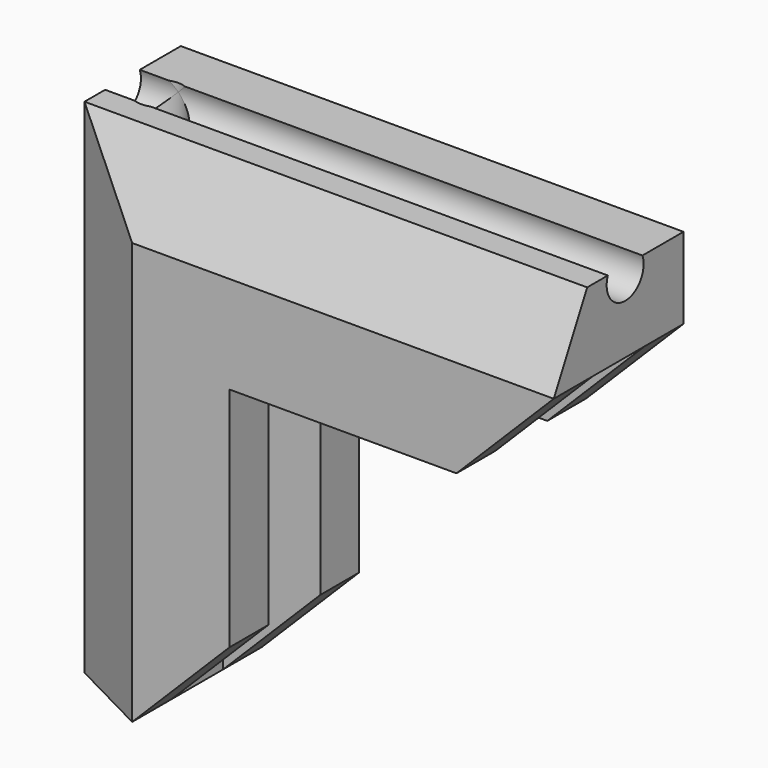
from build123d import *

# Parameters (mm, degrees)
F1_DEPTH      = 20
F2_W          = 7
F2_H          = 20
F3_DEPTH      = 2
F5_DEPTH      = 6
F6_W          = 3
F6_H          = 6
F7_DEPTH      = 25
F8_DEPTH      = 3
F12_DEPTH     = 2
F13_DEPTH     = 11
F14_T4_DEPTH  = 29
F14_T10_DEPTH = 28
F14_T17_DEPTH = 38.2867319519
F14_T24_DEPTH = 39.2867319519
F15_T1_DEPTH  = 61.1449358039
F15_T3_DEPTH  = 60.1449358039
F16_DEPTH     = 1
F17_SIZE      = 6
F20_D         = 2.85
F20_ON_F18_D  = 2.85


# Not quite as in the source:
# - a fillet or chamfer that OpenCascade refuses, or shapes differently, is made with other operations: its cross-section is extruded or revolved along the edge and cut away or added


with BuildPart() as f1:
    # F0 (on Top) → F1 (new body)
    with BuildSketch(Plane.XY):
        Polygon((-3.1551690071, 9.1141472052), (-12.1551690071, 9.1141472052), (-12.1551690071, -0.8858527948), (-3.1551690071, -0.8858527948), (-3.1551690071, 2.1141472052), (-9.1551690071, 2.1141472052), (-9.1551690071, 6.1141472052), (-3.1551690071, 6.1141472052), align=None)
    extrude(amount=F1_DEPTH)

    # F2 (on face) → F3 (join)
    with BuildSketch(Plane(origin=(-12.1551690071, 0, 0), x_dir=(0, -1, 0), z_dir=(-1, 0, 0))):
        with Locations((-5.6141472052, 10)):
            Rectangle(F2_W, F2_H)
    extrude(amount=F3_DEPTH)

    # F4 (on face) → F5 (join)
    with BuildSketch(Plane.XY.offset(20)):
        Polygon((-12.1345976368, 9.1141472052), (-12.1551690071, 2.1141472052), (-12.1551690071, -0.8858527948), (-9.1551690071, -0.8858527948), (-9.1551690071, 2.1141472052), (-9.1551690071, 6.1141472052), (-9.1551690071, 9.1141472052), align=None)
    extrude(amount=F5_DEPTH)

    # F6 (on face) → F7 (join)
    with BuildSketch(Plane.YZ.offset(-9.1551690071)):
        with Locations((7.6141472052, 23)):
            Rectangle(F6_W, F6_H)
        with Locations((0.6141472052, 23)):
            Rectangle(F6_W, F6_H)
        Polygon((-0.8858527948, 26), (2.1141472052, 26), (6.1141472052, 26), (9.1141472052, 26), (9.1141472052, 29), (-0.8858527948, 29), align=None)
    extrude(amount=F7_DEPTH)

    # F8 (add): a face of the model
    f8_faces = [f1.faces().sort_by_distance(p)[0] for p in [
        (-10.6515768532, 4.1077318265, 26),
    ]]
    extrude(f8_faces, amount=F8_DEPTH)

    # F9: union 

    # F10: union 

    # F11 (on face) → F12 (join)
    with BuildSketch(Plane.XY.offset(29)):
        Polygon((-12.1345976368, 9.1141472052), (-12.1551690071, 2.1141472052), (15.8448309929, 2.1141472052), (15.8448309929, 9.1141472052), align=None)
    extrude(amount=F12_DEPTH)

    # F4 (on face) → F13 (join)
    with BuildSketch(Plane.XY.offset(20)):
        Polygon((-14.1551690071, 2.1141472052), (-12.1551690071, 2.1141472052), (-12.1345976368, 9.1141472052), (-14.1551690071, 9.1141472052), align=None)
    extrude(amount=F13_DEPTH)

    # F14: chamfer of 4 on 2 edges, made by hand


with BuildPart() as f14_tool2:
    # F14_s3 → F14_t4 (new body)
    with BuildSketch(Plane.XY):
        Polygon((-12.1551690071, -1.8858527948), (-16.1551690071, 2.1141472052), (-12.1551690071, 2.1141472052), align=None)
    extrude(amount=F14_T4_DEPTH)

    split(bisect_by=Plane.XZ.offset(0.8858527948), keep=Keep.BOTTOM)

    split(bisect_by=Plane.YZ.offset(-14.1551690071), keep=Keep.TOP)


with BuildPart() as f1_1:
    add(f1.part)

    # F14_t1: union F14_tool2
    add(f14_tool2.part)


with BuildPart() as f14_tool8:
    # F14_s9 → F14_t10 (new body)
    with BuildSketch(Plane.YZ.offset(-12.1551690071)):
        Polygon((-1.8858527948, 29), (2.1141472052, 33), (2.1141472052, 29), align=None)
    extrude(amount=F14_T10_DEPTH)

    split(bisect_by=Plane.XZ.offset(0.8858527948), keep=Keep.BOTTOM)

    split(bisect_by=Plane.XY.offset(31), keep=Keep.BOTTOM)


with BuildPart() as f1_2:
    add(f1_1.part)

    # F14_t7: union F14_tool8
    add(f14_tool8.part)


with BuildPart() as f14_tool15:
    # F14_s16 → F14_t17 (new body)
    with BuildSketch(Plane.YZ.offset(-22.4419009589)):
        Polygon((-1.8858527948, 29), (2.1141472052, 33), (2.1141472052, 29), align=None)
    extrude(amount=F14_T17_DEPTH)

    split(bisect_by=Plane.XZ.offset(0.8858527948), keep=Keep.BOTTOM)

    split(bisect_by=Plane.YZ.offset(-12.1551690071), keep=Keep.BOTTOM)

    split(bisect_by=Plane.YZ.offset(-14.1551690071), keep=Keep.TOP)

    split(bisect_by=Plane.XY.offset(31), keep=Keep.BOTTOM)


with BuildPart() as f14_tool22:
    # F14_s23 → F14_t24 (new body)
    with BuildSketch(Plane.XY):
        Polygon((-12.1551690071, -1.8858527948), (-16.1551690071, 2.1141472052), (-12.1551690071, 2.1141472052), align=None)
    extrude(amount=F14_T24_DEPTH)

    split(bisect_by=Plane.XZ.offset(0.8858527948), keep=Keep.BOTTOM)

    split(bisect_by=Plane.XY.offset(29), keep=Keep.TOP)

    split(bisect_by=Plane.YZ.offset(-14.1551690071), keep=Keep.TOP)

    split(bisect_by=Plane.XY.offset(31), keep=Keep.BOTTOM)


with BuildPart() as f14_tool15_1:
    add(f14_tool15.part)

    # F14_t29: intersect F14_tool22
    add(f14_tool22.part, mode=Mode.INTERSECT)


with BuildPart() as f1_3:
    add(f1_2.part)

    # F14_t13: union F14_tool15
    add(f14_tool15_1.part)

    # F15: chamfer of 4 x 6 on 2 edges, made by hand

    # F15_s2 → F15_t1 (cut)
    with BuildSketch(Plane.XY.offset(-15.5724679019)):
        Polygon((-9.1551690071, -0.8858527948), (-17.3978096942, 3.3567878923), (-13.1551690071, -0.8858527948), align=None)
    extrude(amount=F15_T1_DEPTH, mode=Mode.SUBTRACT)

    # F15_s4 → F15_t3 (cut)
    with BuildSketch(Plane.YZ.offset(-28.7276369091)):
        Polygon((-0.8858527948, 26), (3.3567878923, 34.2426406871), (-0.8858527948, 30), align=None)
    extrude(amount=F15_T3_DEPTH, mode=Mode.SUBTRACT)

    # F16 (add): a face of the model
    f16_faces = [f1_3.faces().sort_by_distance(p)[0] for p in [
        (15.8448309929, 6.2628078927, 23),
    ]]
    extrude(f16_faces, amount=F16_DEPTH)

    # F17
    f17_edges = [f1_3.edges().sort_by_distance(p)[0] for p in [
        (-3.155169, 0.614147, 0),
        (-3.155169, 7.614147, 0),
        (16.844831, 0.614147, 20),
        (16.844831, 7.614147, 20),
    ]]
    chamfer(f17_edges, length=F17_SIZE)

    # F20 (through all)
    with Locations(Plane(origin=(0, 0, 0), x_dir=(1, 0, 0), z_dir=(0, 0, -1))):
        with Locations((-11.8551690071, -4.6141472052)):
            Hole(F20_D / 2)

    # F20 on F18 (through all)
    with Locations(Plane.YZ.offset(16.8448309929)):
        with Locations((4.6141472052, 30.5)):
            Hole(F20_ON_F18_D / 2)


solid = f1_3.part
